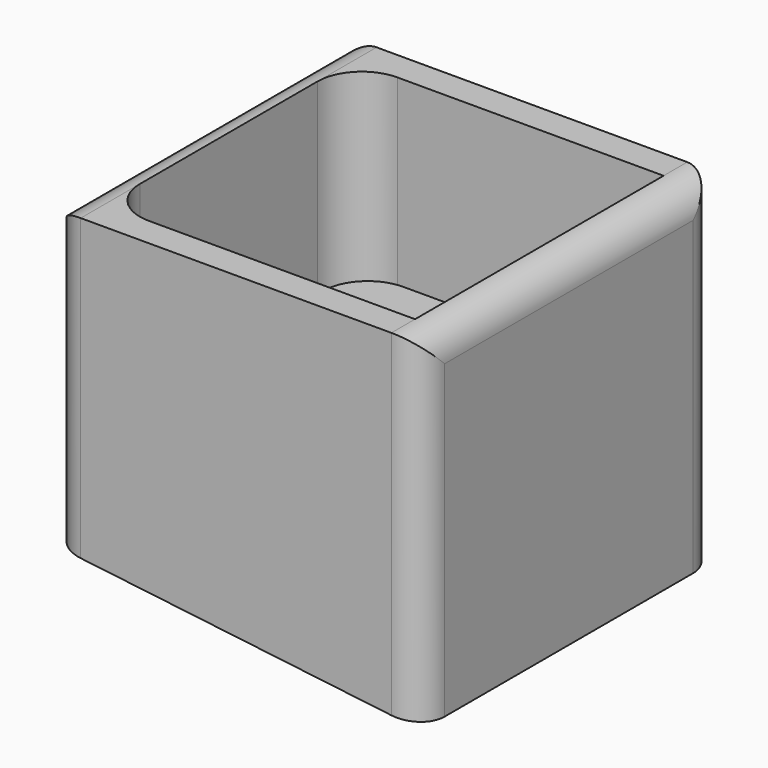
from build123d import *

# Parameters (mm, degrees)
F0_W     = 25
F0_H     = 25
F0_W_2   = 21
F0_H_2   = 21
F1_DEPTH = 23
F0_W_3   = 17
F0_H_3   = 17
F2_DEPTH = 5
F0_W_4   = 11
F0_H_4   = 11
F3_DEPTH = 12
F4_DEPTH = 3
F5_DEPTH = 1
F7_DEPTH = 25
F8_R     = 1.99999
F9_R     = 3


# Not quite as in the source:
# - a fillet or chamfer is up to 0.001 mm smaller than in the source, because OpenCascade refuses the exact size


with BuildPart() as f1:
    # F0 (on Top) → F1 (new body)
    with BuildSketch(Plane.XY):
        with Locations((12.5, -12.5)):
            Rectangle(F0_W, F0_H)
        with Locations((12.5, -12.5)):
            Rectangle(F0_W_2, F0_H_2, mode=Mode.SUBTRACT)
    extrude(amount=F1_DEPTH)

    # F0 (on Top) → F2 (join)
    with BuildSketch(Plane.XY):
        with Locations((12.5, -12.5)):
            Rectangle(F0_W_2, F0_H_2)
        with Locations((12.5, -12.5)):
            Rectangle(F0_W_3, F0_H_3, mode=Mode.SUBTRACT)
    extrude(amount=F2_DEPTH)

    # F0 (on Top) → F3 (join)
    with BuildSketch(Plane.XY):
        with Locations((12.5, -12.5)):
            Rectangle(F0_W_3, F0_H_3)
        with Locations((12.5, -12.5)):
            Rectangle(F0_W_4, F0_H_4, mode=Mode.SUBTRACT)
        with Locations((12.5, -12.5)):
            Rectangle(F0_W_4, F0_H_4)
    extrude(amount=F3_DEPTH)

    # F0 (on Top) → F4 (cut)
    with BuildSketch(Plane.XY):
        with Locations((12.5, -12.5)):
            Rectangle(F0_W_4, F0_H_4)
    extrude(amount=F4_DEPTH, mode=Mode.SUBTRACT)

    # F0 (on Top) → F5 (cut)
    with BuildSketch(Plane.XY):
        with Locations((12.5, -12.5)):
            Rectangle(F0_W_2, F0_H_2)
        with Locations((12.5, -12.5)):
            Rectangle(F0_W_3, F0_H_3, mode=Mode.SUBTRACT)
    extrude(amount=F5_DEPTH, mode=Mode.SUBTRACT)

    # F6 (on face) → F7 (cut, through all)
    with BuildSketch(Plane.XZ.offset(25)):
        Polygon((25, 0), (0, 3), (0, 0), align=None)
    extrude(amount=-F7_DEPTH, mode=Mode.SUBTRACT)

    # F8 (radius 2 in the source; OpenCascade refuses exactly that, so slightly less here)
    f8_edges = [f1.edges().sort_by_distance(p)[0] for p in [
        (25, -25, 11.5),
        (0, -25, 13),
        (0, 0, 13),
        (25, 0, 11.5),
        (0, -12.5, 23),
        (25, -12.5, 23),
    ]]
    fillet(f8_edges, radius=F8_R)

    # F9
    f9_edges = [f1.edges().sort_by_distance(p)[0] for p in [
        (2, -2, 14),
        (4, -4, 8.5),
        (21, -4, 8.5),
        (21, -21, 8.5),
        (4, -21, 8.5),
        (2, -23, 14),
    ]]
    fillet(f9_edges, radius=F9_R)


solid = f1.part
